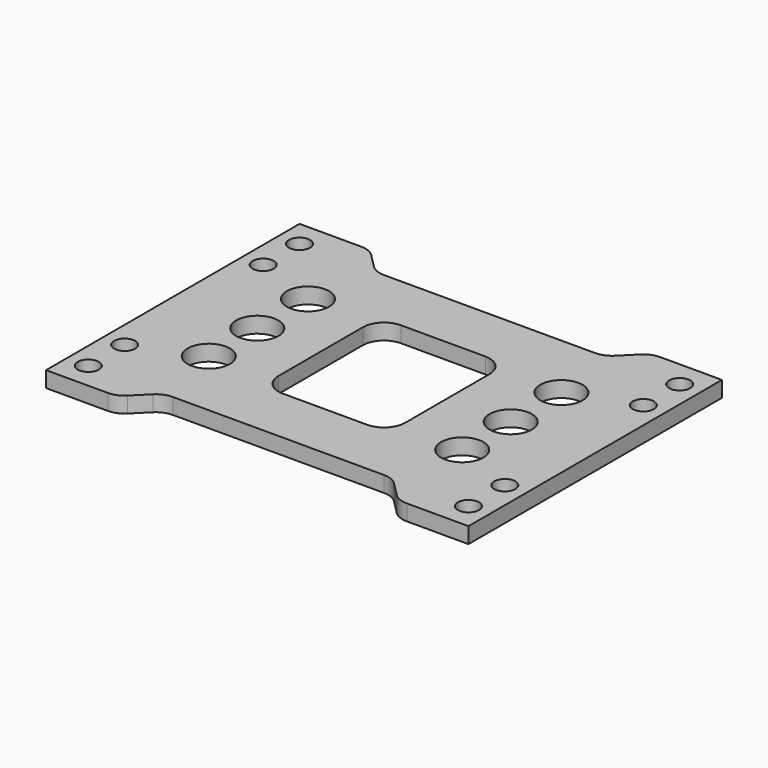
from build123d import *

# Parameters (mm, degrees)
F0_R     = 1
F0_R_2   = 2
F1_DEPTH = 1.5
F2_SCALE = 10


# Not quite as in the source:
# - ends of sketch curves that miss each other by under 0.0002 mm in the source are joined


with BuildPart() as f1:
    # F0 (on Top) → F1 (new body)
    with BuildSketch(Plane.XY):
        with BuildLine():
            ThreePointArc((14.156854, 15), (13.3914871353, 14.847759065), (12.7426404376, 14.4142135624))
            Line((12.7426404376, 14.4142135624), (11.414213, 13.085786))
            ThreePointArc((11.414213, 13.085786), (10.7653665381, 12.6522407997), (10, 12.5))
            Line((10, 12.5), (-10, 12.5))
            ThreePointArc((-10, 12.5), (-10.7653668647, 12.652240935), (-11.4142135624, 13.0857864376))
            Line((-11.4142135624, 13.0857864376), (-12.742641, 14.414213))
            ThreePointArc((-12.742641, 14.414213), (-13.3914871353, 14.847759065), (-14.156854, 15))
            Line((-14.156854, 15), (-20, 15))
            Line((-20, 15), (-20, -15))
            Line((-20, -15), (-14.156854, -15))
            ThreePointArc((-14.156854, -15), (-13.3914874619, -14.8477592003), (-12.7426409376, -14.4142140624))
            Line((-12.7426409376, -14.4142140624), (-11.414214, -13.085787))
            ThreePointArc((-11.414214, -13.085787), (-10.7653671914, -12.6522410703), (-10, -12.5))
            Line((-10, -12.5), (10, -12.5))
            ThreePointArc((10, -12.5), (10.7653668647, -12.652240935), (11.4142135624, -13.0857864376))
            Line((11.4142135624, -13.0857864376), (12.742641, -14.414214))
            ThreePointArc((12.742641, -14.414214), (13.3914874619, -14.8477592003), (14.156854, -15))
            Line((14.156854, -15), (20, -15))
            Line((20, -15), (20, 15))
            Line((20, 15), (14.156854, 15))
        make_face()
        with Locations((-18, -12.5)):
            Circle(F0_R, mode=Mode.SUBTRACT)
        with Locations((-18, -8.2)):
            Circle(F0_R, mode=Mode.SUBTRACT)
        with Locations((-12, -5.744006)):
            Circle(F0_R_2, mode=Mode.SUBTRACT)
        with Locations((18, -12.5)):
            Circle(F0_R, mode=Mode.SUBTRACT)
        with Locations((18, -8.2)):
            Circle(F0_R, mode=Mode.SUBTRACT)
        with Locations((12, -5.744006)):
            Circle(F0_R_2, mode=Mode.SUBTRACT)
        with Locations((-12, 0)):
            Circle(F0_R_2, mode=Mode.SUBTRACT)
        with Locations((-12, 6)):
            Circle(F0_R_2, mode=Mode.SUBTRACT)
        with Locations((-18, 8.2)):
            Circle(F0_R, mode=Mode.SUBTRACT)
        with Locations((-18, 12.5)):
            Circle(F0_R, mode=Mode.SUBTRACT)
        with BuildLine():
            ThreePointArc((-6, 5), (-5.4142135624, 6.4142135624), (-4, 7))
            Line((-4, 7), (4, 7))
            ThreePointArc((4, 7), (5.4142135624, 6.4142135624), (6, 5))
            Line((6, 5), (6, -5))
            ThreePointArc((6, -5), (5.4142135624, -6.4142135624), (4, -7))
            Line((4, -7), (-4, -7))
            ThreePointArc((-4, -7), (-5.4142135624, -6.4142135624), (-6, -5))
            Line((-6, -5), (-6, 5))
        make_face(mode=Mode.SUBTRACT)
        with Locations((12, 0)):
            Circle(F0_R_2, mode=Mode.SUBTRACT)
        with Locations((12, 6)):
            Circle(F0_R_2, mode=Mode.SUBTRACT)
        with Locations((18, 8.2)):
            Circle(F0_R, mode=Mode.SUBTRACT)
        with Locations((18, 12.5)):
            Circle(F0_R, mode=Mode.SUBTRACT)
    extrude(amount=F1_DEPTH)


with BuildPart() as f1_1:
    # F2: moved
    add(f1.part.scale(F2_SCALE).moved(Location((180, 135, -13.5))))


solid = f1_1.part
